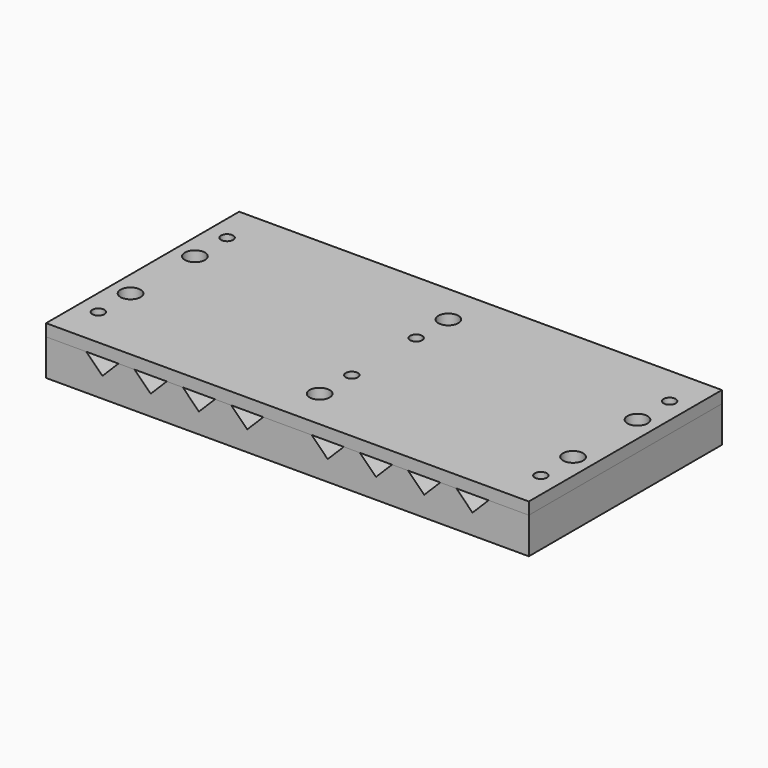
from build123d import *

# Parameters (mm, degrees)
F0_W     = 120
F0_H     = 60
F1_DEPTH = 5
F3_DEPTH = 60
F4_D     = 5
F5_D     = 5
F6_D     = 3
F7_W     = 54
F7_H     = 60
F7_W_2   = 12
F7_R     = 2.5
F7_R_2   = 1.5
F8_DEPTH = 3
F9_D     = 3
F10_D    = 5


with BuildPart() as f1:
    # F0 (on Top) → F1 (new body)
    with BuildSketch(Plane.XY):
        with Locations((60, 30)):
            Rectangle(F0_W, F0_H)
    extrude(amount=F1_DEPTH)

    # F2 (on face) → F3 (join)
    with BuildSketch(Plane.XZ):
        Polygon((106, 5), (120, 5), (120, 9), (110, 9), align=None)
        Polygon((94, 5), (106, 5), (102, 9), (98, 9), align=None)
        Polygon((82, 5), (94, 5), (90, 9), (86, 9), align=None)
        Polygon((70, 5), (82, 5), (78, 9), (74, 9), align=None)
        Polygon((54, 9), (50, 5), (70, 5), (66, 9), align=None)
        Polygon((42, 9), (38, 5), (50, 5), (46, 9), align=None)
        Polygon((30, 9), (26, 5), (38, 5), (34, 9), align=None)
        Polygon((18, 9), (14, 5), (26, 5), (22, 9), align=None)
        Polygon((0, 9), (0, 5), (14, 5), (10, 9), align=None)
    extrude(amount=-F3_DEPTH)

    # F4 (through all)
    with Locations(Plane(origin=(0, 0, 0), x_dir=(1, 0, 0), z_dir=(0, 0, -1))):
        with Locations((115, -20), (115, -40), (5, -20), (5, -40)):
            Hole(F4_D / 2)

    # F5 (through all)
    with Locations(Plane(origin=(0, 0, 0), x_dir=(1, 0, 0), z_dir=(0, 0, -1))):
        with Locations((60, -50), (60, -10)):
            Hole(F5_D / 2)

    # F6 (through all)
    with Locations(Plane(origin=(0, 0, 0), x_dir=(1, 0, 0), z_dir=(0, 0, -1))):
        with Locations((5, -50), (5, -10), (60, -40), (60, -20), (115, -10), (115, -50)):
            Hole(F6_D / 2)


with BuildPart() as f8:
    # F7 (on face) → F8 (new body)
    with BuildSketch(Plane.XY.offset(9)):
        with Locations((27, 30)):
            Rectangle(F7_W, F7_H)
        with Locations((93, 30)):
            Rectangle(F7_W, F7_H)
        with Locations((60, 30)):
            Rectangle(F7_W_2, F7_H)
        with Locations((60, 10)):
            Circle(F7_R, mode=Mode.SUBTRACT)
        with Locations((60, 20)):
            Circle(F7_R_2, mode=Mode.SUBTRACT)
        with Locations((60, 40)):
            Circle(F7_R_2, mode=Mode.SUBTRACT)
        with Locations((60, 50)):
            Circle(F7_R, mode=Mode.SUBTRACT)
    extrude(amount=F8_DEPTH)

    # F9 (through all)
    with Locations(Plane(origin=(0, 0, 0), x_dir=(1, 0, 0), z_dir=(0, 0, -1))):
        with Locations((115, -10), (115, -50), (60, -40), (60, -20), (5, -10), (5, -50)):
            Hole(F9_D / 2)

    # F10 (through all)
    with Locations(Plane(origin=(0, 0, 0), x_dir=(1, 0, 0), z_dir=(0, 0, -1))):
        with Locations((115, -20), (115, -40), (60, -50), (60, -10), (5, -20), (5, -40)):
            Hole(F10_D / 2)


solid = Compound([f1.part, f8.part])
